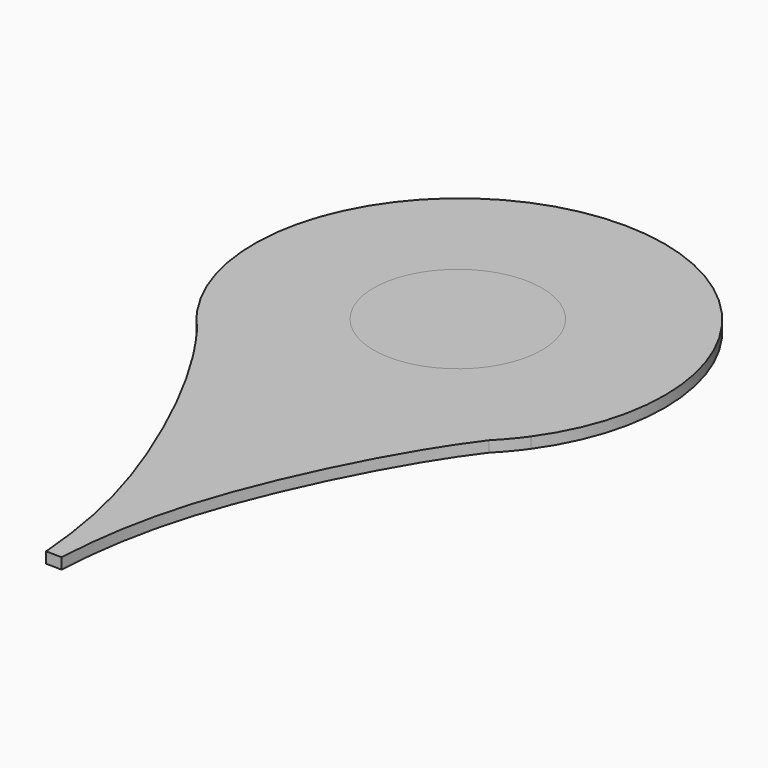
from build123d import *

# Parameters (mm, degrees)
F2_R     = 23.0897028216
F3_DEPTH = 3
F0_R     = 23.0897028216
F4_DEPTH = 3


# Not quite as in the source:
# - the dataset's text gives a spline's control points without its knots; the knots are read off the source's solid


with BuildPart() as f3:
    # F2 (on face) → F3 (new body)
    with BuildSketch(Plane.XY):
        with BuildLine():
            add(Edge.make_bspline(
                [(24.4357683195, 13.7704961499), (26.4004851942, 16.3478745215), (28.3743311543, 18.6940959772), (30.3351804614, 20.7458790392)],
                knots=[0.9099263798, 0.9099263798, 0.9099263798, 0.9099263798, 1, 1, 1, 1], degree=3))
            ThreePointArc((24.4357683195, 13.7704961499), (27.527158464, 17.1383586537), (30.3351804614, 20.7458790392))
        make_face()
        with BuildLine():
            add(Edge.make_bspline(
                [(-13.1657877937, -85.7971683145), (-12.124221772, -65.5360594392), (-4.0500259711, -34.9286832493), (15.3721634866, 1.8805697355), (24.4357683195, 13.7704961499)],
                knots=[0, 0, 0, 0, 0.4943999951, 0.9099263798, 0.9099263798, 0.9099263798, 0.9099263798], degree=3))
            add(Edge.make_bspline(
                [(24.4357683195, 13.7704961499), (26.4004851942, 16.3478745215), (28.3743311543, 18.6940959772), (30.3351804614, 20.7458790392)],
                knots=[0.9099263798, 0.9099263798, 0.9099263798, 0.9099263798, 1, 1, 1, 1], degree=3))
            ThreePointArc((30.3351804614, 20.7458790392), (-14.8805945591, 109.8132814972), (-61.9512721896, 21.7120908201))
            add(Edge.make_bspline(
                [(-56.8019096606, 15.2559147606), (-58.4646697135, 17.4695314371), (-60.1806042841, 19.6250655082), (-61.9512721896, 21.7120908201)],
                knots=[0.9292469814, 0.9292469814, 0.9292469814, 0.9292469814, 1, 1, 1, 1], degree=3))
            add(Edge.make_bspline(
                [(-17.4547079951, -85.7477933168), (-19.0374422117, -64.7392000389), (-29.0853821507, -31.9599274574), (-46.6665856361, 1.7628540852), (-56.8019096606, 15.2559147606)],
                knots=[0, 0, 0, 0, 0.497973228, 0.9292469814, 0.9292469814, 0.9292469814, 0.9292469814], degree=3))
            Line((-17.4547079951, -85.7477933168), (-13.1657877937, -85.7971683145))
        make_face()
        with Locations((-15.9126216176, 53.508865199)):
            Circle(F2_R, mode=Mode.SUBTRACT)
        with BuildLine():
            add(Edge.make_bspline(
                [(-56.8019096606, 15.2559147606), (-58.4646697135, 17.4695314371), (-60.1806042841, 19.6250655082), (-61.9512721896, 21.7120908201)],
                knots=[0.9292469814, 0.9292469814, 0.9292469814, 0.9292469814, 1, 1, 1, 1], degree=3))
            ThreePointArc((-61.9512721896, 21.7120908201), (-59.4950986731, 18.3894825431), (-56.8019096606, 15.2559147606))
        make_face()
    extrude(amount=F3_DEPTH)


with BuildPart() as f4:
    # F0 (on Top) → F4 (new body)
    with BuildSketch(Plane.XY):
        with Locations((-15.9126216176, 53.508865199)):
            Circle(F0_R)
    extrude(amount=F4_DEPTH)


solid = Compound([f3.part, f4.part])
